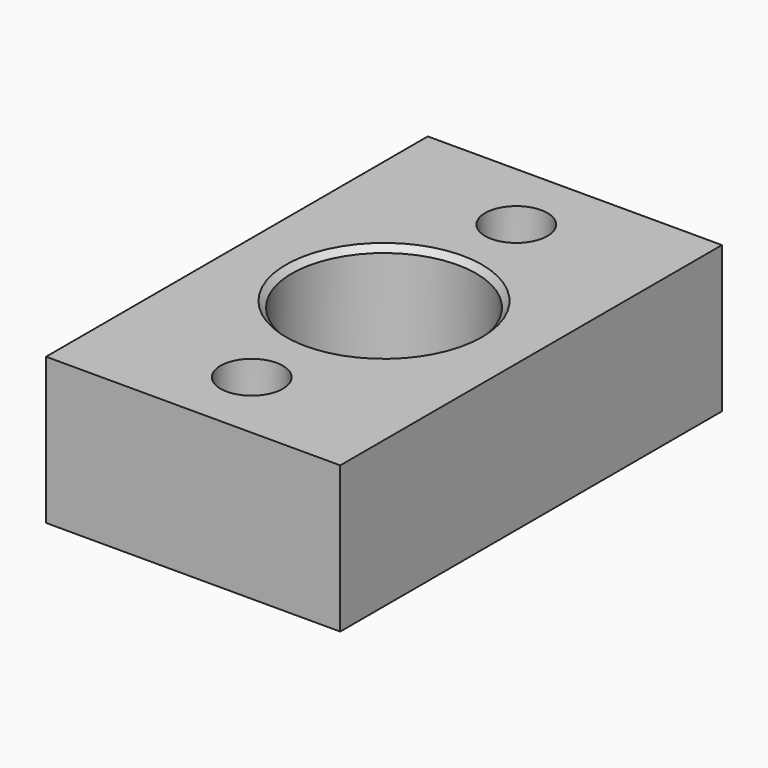
from build123d import *

# Parameters (mm, degrees)
F0_W     = 12.7625
F0_H     = 20.7
F0_R     = 1.35255
F0_R_2   = 4
F1_DEPTH = 6.35
F2_SIZE  = 0.254


# Not quite as in the source:
# - a feature names something its author has since deleted; it is built from what else it names


with BuildPart() as f1:
    # F0 (on Top) → F1 (new body)
    with BuildSketch(Plane.XY):
        Rectangle(F0_W, F0_H)
        with Locations((0, -7.175)):
            Circle(F0_R, mode=Mode.SUBTRACT)
        Circle(F0_R_2, mode=Mode.SUBTRACT)
        with Locations((0, 7.175)):
            Circle(F0_R, mode=Mode.SUBTRACT)
    extrude(amount=F1_DEPTH)

    # F2
    f2_edges = [f1.edges().sort_by_distance(p)[0] for p in [
        (-4, 0, 6.35),
    ]]
    chamfer(f2_edges, length=F2_SIZE)


solid = f1.part
